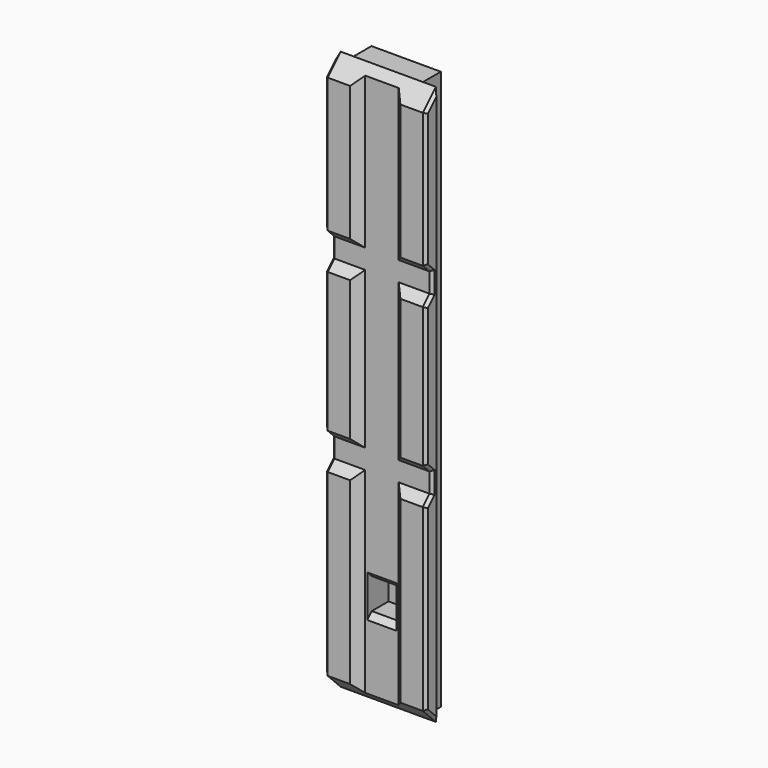
from build123d import *

# Parameters (mm, degrees)
F1_DEPTH      = 100
F3_DEPTH      = 25
F3_DEPTH_BACK = 25
F4_SIZE       = 2.90999
F5_SIZE       = 2.90999
F7_DEPTH      = 6.25
F8_SIZE       = 1
F9_C1_SIZE    = 0.5
F9_C2_SIZE    = 0.5
F9_C3_SIZE    = 0.5
F9_C4_SIZE    = 0.5
F9_C5_SIZE    = 0.5
F9_C6_SIZE    = 0.5
F9_C7_SIZE    = 0.5
F9_C8_SIZE    = 0.5
F9_C9_SIZE    = 0.5
F9_C10_SIZE   = 0.5
F9_C11_SIZE   = 0.5
F9_C12_SIZE   = 0.5
F9_C13_SIZE   = 0.5
F9_C14_SIZE   = 0.5
F9_C15_SIZE   = 0.5
F9_C16_SIZE   = 0.5
F9_C17_SIZE   = 0.5
F9_C18_SIZE   = 0.5
F9_C19_SIZE   = 0.5
F9_C20_SIZE   = 0.5
F9_C21_SIZE   = 0.5
F9_C22_SIZE   = 0.5
F9_C23_SIZE   = 0.5
F9_C24_SIZE   = 0.5


# Not quite as in the source:
# - a fillet or chamfer is up to 0.001 mm smaller than in the source, because OpenCascade refuses the exact size


with BuildPart() as f1:
    # F0 (on Top) → F1 (new body)
    with BuildSketch(Plane.XY):
        Polygon((0, 2.91), (0, 0), (4.5, 0), (6, 1.5), (12, 1.5), (13.5, 0), (18, 0), (18, 2.91), (15.2, 2.91), (15.2, 6.91), (2.8, 6.91), (2.8, 2.91), align=None)
    extrude(amount=F1_DEPTH)

    # F2 (on Right) → F3 (cut, two sides)
    with BuildSketch(Plane.YZ) as f3_sk:
        Polygon((-0.9837878169, 0), (0, 0), (0, 35), (1.5, 36.5), (1.5, 40), (0, 41.5), (0, 66.5), (1.5, 68), (1.5, 71.5), (0, 73), (0, 100.0014618039), (-0.9837878169, 100.0014618039), align=None)
    extrude(amount=-F3_DEPTH, mode=Mode.SUBTRACT)
    extrude(f3_sk.sketch, amount=F3_DEPTH_BACK, mode=Mode.SUBTRACT)

    # F4 (size 2.91 in the source; OpenCascade refuses exactly that, so slightly less here)
    f4_edges = [f1.edges().sort_by_distance(p)[0] for p in [
        (2.25, 0, 0),
    ]]
    chamfer(f4_edges, length=F4_SIZE)

    # F5 (size 2.91 in the source; OpenCascade refuses exactly that, so slightly less here)
    f5_edges = [f1.edges().sort_by_distance(p)[0] for p in [
        (15.75, 0, 100),
    ]]
    chamfer(f5_edges, length=F5_SIZE)

    # F6 (on Front) → F7 (cut)
    with BuildSketch(Plane.XZ):
        Polygon((6.375, 14), (9, 14), (11.625, 14), (11.625, 19.5), (6.375, 19.5), align=None)
    extrude(amount=-F7_DEPTH, mode=Mode.SUBTRACT)

    # F8
    f8_edges = [f1.edges().sort_by_distance(p)[0] for p in [
        (9, 1.5, 14),
        (9, 1.5, 19.5),
    ]]
    chamfer(f8_edges, length=F8_SIZE)

    # F9: chamfer of 0.5 on 28 edges, made by hand

    # F9_c1
    f9_c1_edges = [f1.edges().sort_by_distance(p)[0] for p in [
        (18, 2.91, 50),
    ]]
    chamfer(f9_c1_edges, length=F9_C1_SIZE)

    # F9_c2
    f9_c2_edges = [f1.edges().sort_by_distance(p)[0] for p in [
        (0, 2.91, 50),
    ]]
    chamfer(f9_c2_edges, length=F9_C2_SIZE)

    # F9_c3
    f9_c3_edges = [f1.edges().sort_by_distance(p)[0] for p in [
        (18, 0, 18.954995),
    ]]
    chamfer(f9_c3_edges, length=F9_C3_SIZE)

    # F9_c4
    f9_c4_edges = [f1.edges().sort_by_distance(p)[0] for p in [
        (0, 0, 18.954995),
    ]]
    chamfer(f9_c4_edges, length=F9_C4_SIZE)

    # F9_c5
    f9_c5_edges = [f1.edges().sort_by_distance(p)[0] for p in [
        (18, 0, 54),
    ]]
    chamfer(f9_c5_edges, length=F9_C5_SIZE)

    # F9_c6
    f9_c6_edges = [f1.edges().sort_by_distance(p)[0] for p in [
        (0, 0, 54),
    ]]
    chamfer(f9_c6_edges, length=F9_C6_SIZE)

    # F9_c7
    f9_c7_edges = [f1.edges().sort_by_distance(p)[0] for p in [
        (0, 0, 85.045005),
    ]]
    chamfer(f9_c7_edges, length=F9_C7_SIZE)

    # F9_c8
    f9_c8_edges = [f1.edges().sort_by_distance(p)[0] for p in [
        (18, 0, 85.045005),
    ]]
    chamfer(f9_c8_edges, length=F9_C8_SIZE)

    # F9_c9
    f9_c9_edges = [f1.edges().sort_by_distance(p)[0] for p in [
        (18, 1.455, 1.45499),
    ]]
    chamfer(f9_c9_edges, length=F9_C9_SIZE)

    # F9_c10
    f9_c10_edges = [f1.edges().sort_by_distance(p)[0] for p in [
        (0, 1.455, 1.45499),
    ]]
    chamfer(f9_c10_edges, length=F9_C10_SIZE)

    # F9_c11
    f9_c11_edges = [f1.edges().sort_by_distance(p)[0] for p in [
        (18, 1.455, 98.54501),
    ]]
    chamfer(f9_c11_edges, length=F9_C11_SIZE)

    # F9_c12
    f9_c12_edges = [f1.edges().sort_by_distance(p)[0] for p in [
        (0, 1.455, 98.54501),
    ]]
    chamfer(f9_c12_edges, length=F9_C12_SIZE)

    # F9_c13
    f9_c13_edges = [f1.edges().sort_by_distance(p)[0] for p in [
        (18, 1.5, 69.75),
    ]]
    chamfer(f9_c13_edges, length=F9_C13_SIZE)

    # F9_c14
    f9_c14_edges = [f1.edges().sort_by_distance(p)[0] for p in [
        (0, 1.5, 69.75),
    ]]
    chamfer(f9_c14_edges, length=F9_C14_SIZE)

    # F9_c15
    f9_c15_edges = [f1.edges().sort_by_distance(p)[0] for p in [
        (18, 1.5, 38.25),
    ]]
    chamfer(f9_c15_edges, length=F9_C15_SIZE)

    # F9_c16
    f9_c16_edges = [f1.edges().sort_by_distance(p)[0] for p in [
        (0, 1.5, 38.25),
    ]]
    chamfer(f9_c16_edges, length=F9_C16_SIZE)

    # F9_c17
    f9_c17_edges = [f1.edges().sort_by_distance(p)[0] for p in [
        (18, 1, 36),
    ]]
    chamfer(f9_c17_edges, length=F9_C17_SIZE)

    # F9_c18
    f9_c18_edges = [f1.edges().sort_by_distance(p)[0] for p in [
        (18, 1, 40.5),
    ]]
    chamfer(f9_c18_edges, length=F9_C18_SIZE)

    # F9_c19
    f9_c19_edges = [f1.edges().sort_by_distance(p)[0] for p in [
        (0, 1, 72),
    ]]
    chamfer(f9_c19_edges, length=F9_C19_SIZE)

    # F9_c20
    f9_c20_edges = [f1.edges().sort_by_distance(p)[0] for p in [
        (18, 1, 72),
    ]]
    chamfer(f9_c20_edges, length=F9_C20_SIZE)

    # F9_c21
    f9_c21_edges = [f1.edges().sort_by_distance(p)[0] for p in [
        (18, 1, 67.5),
    ]]
    chamfer(f9_c21_edges, length=F9_C21_SIZE)

    # F9_c22
    f9_c22_edges = [f1.edges().sort_by_distance(p)[0] for p in [
        (0, 1, 36),
    ]]
    chamfer(f9_c22_edges, length=F9_C22_SIZE)

    # F9_c23
    f9_c23_edges = [f1.edges().sort_by_distance(p)[0] for p in [
        (0, 1, 40.5),
    ]]
    chamfer(f9_c23_edges, length=F9_C23_SIZE)

    # F9_c24
    f9_c24_edges = [f1.edges().sort_by_distance(p)[0] for p in [
        (0, 1, 67.5),
    ]]
    chamfer(f9_c24_edges, length=F9_C24_SIZE)


solid = f1.part
